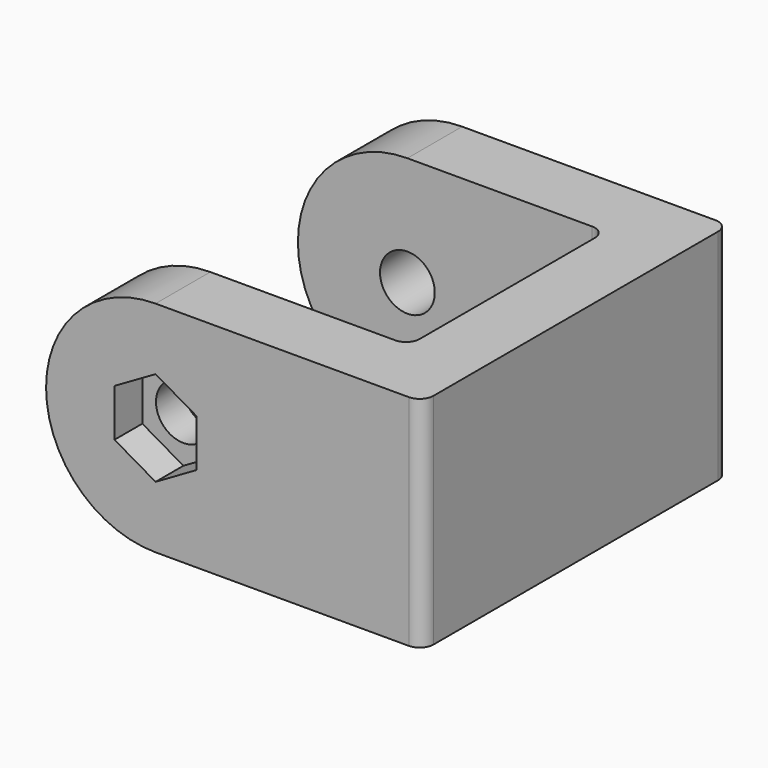
from build123d import *

# Parameters (mm, degrees)
F1_DEPTH = 16
F3_D     = 4
F3_DEPTH = 30
F3_TIP   = 1.2017212381
F4_R     = 1
F5_R     = 7.99999
F6_DEPTH = 2.54


# Not quite as in the source:
# - a fillet or chamfer is up to 0.001 mm smaller than in the source, because OpenCascade refuses the exact size


with BuildPart() as f1:
    # F0 (on Top) → F1 (new body)
    with BuildSketch(Plane.XY):
        Polygon((0, 23), (0, 18), (22.5, 18), (22.5, 0), (0, 0), (0, -5), (27.5, -5), (27.5, 23), align=None)
    extrude(amount=F1_DEPTH)

    # F3
    with Locations(Plane.XZ.offset(5)):
        with Locations((8, 8)):
            Hole(F3_D / 2, depth=F3_DEPTH)
            with Locations((0, 0, -(F3_DEPTH + F3_TIP / 2))):  # 118° drill point
                Cone(0, F3_D / 2, F3_TIP, mode=Mode.SUBTRACT)

    # F4
    f4_edges = [f1.edges().sort_by_distance(p)[0] for p in [
        (22.5, 18, 8),
        (22.5, 0, 8),
        (27.5, -5, 8),
        (27.5, 23, 8),
    ]]
    fillet(f4_edges, radius=F4_R)

    # F5 (radius 8 in the source; OpenCascade refuses exactly that, so slightly less here)
    f5_edges = [f1.edges().sort_by_distance(p)[0] for p in [
        (0, -2.5, 16),
        (0, 20.5, 16),
        (0, -2.5, 0),
        (0, 20.5, 0),
    ]]
    fillet(f5_edges, radius=F5_R)

    # F2 (on face) → F6 (cut)
    with BuildSketch(Plane.XZ.offset(5)):
        Polygon((11, 6.2679491924), (11, 9.7320508076), (8, 11.4641016151), (5, 9.7320508076), (5, 6.2679491924), (8, 4.5358983849), align=None)
    extrude(amount=-F6_DEPTH, mode=Mode.SUBTRACT)


solid = f1.part
